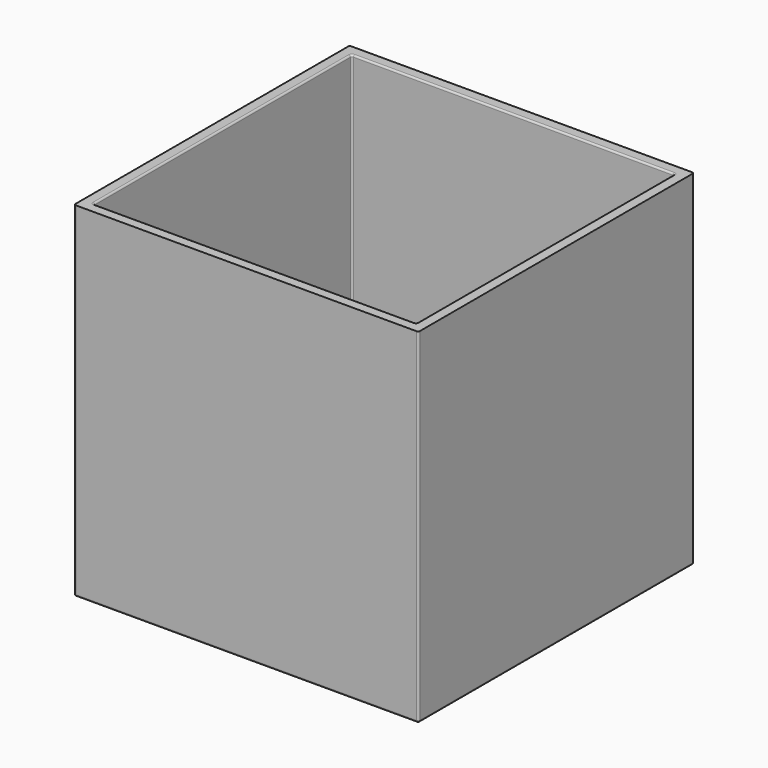
from build123d import *

# Parameters (mm, degrees)
F0_W         = 50.8
F0_H         = 50.8
F1_DEPTH     = 1.5875
F2_W         = 50.8
F2_H         = 50.8
F2_W_2       = 47.625
F2_H_2       = 47.625
F3_DEPTH     = 49.2125
F4_R         = 0.254
F5_TEXT_SIZE = 3.7101570244
F6_DEPTH     = 0.254


# Not quite as in the source:
# - Text() gives the source's letters only with a copy of the font that has no kerning and outlines rounded to 1/6400 em; it was checked with that copy


with BuildPart() as f1:
    # F0 (on Top) → F1 (new body)
    with BuildSketch(Plane.XY):
        Rectangle(F0_W, F0_H)
    extrude(amount=F1_DEPTH)

    # F2 (on face) → F3 (join)
    with BuildSketch(Plane.XY.offset(1.5875)):
        Rectangle(F2_W, F2_H)
        Rectangle(F2_W_2, F2_H_2, mode=Mode.SUBTRACT)
    extrude(amount=F3_DEPTH)

    # F4
    f4_edges = [f1.edges().sort_by_distance(p)[0] for p in [
        (-23.8125, 0, 1.5875),
        (-23.8125, -23.8125, 26.19375),
        (0, -23.8125, 1.5875),
        (-23.8125, 0, 50.8),
        (0, -23.8125, 50.8),
        (0, 23.8125, 1.5875),
        (-23.8125, 23.8125, 26.19375),
        (0, 23.8125, 50.8),
        (23.8125, 23.8125, 26.19375),
        (23.8125, 0, 1.5875),
        (23.8125, 0, 50.8),
        (23.8125, -23.8125, 26.19375),
        (-25.4, -25.4, 25.4),
        (25.4, -25.4, 25.4),
        (25.4, 25.4, 25.4),
        (-25.4, 25.4, 25.4),
        (-25.4, 0, 0),
        (0, -25.4, 0),
        (0, 25.4, 0),
        (25.4, 0, 0),
    ]]
    fillet(f4_edges, radius=F4_R)

    # F5 (on face) → F6 (cut)
    with BuildSketch(Plane(origin=(0, 25.4, 0), x_dir=(-1, 0, 0), z_dir=(0, 1, 0))):
        with Locations((-22.225, 35.4286869425)):
            Text('3-Prong PWM Connectors', F5_TEXT_SIZE, font='Open Sans', text_align=(TextAlign.LEFT, TextAlign.BOTTOM))
    extrude(amount=-F6_DEPTH, mode=Mode.SUBTRACT)


solid = f1.part
